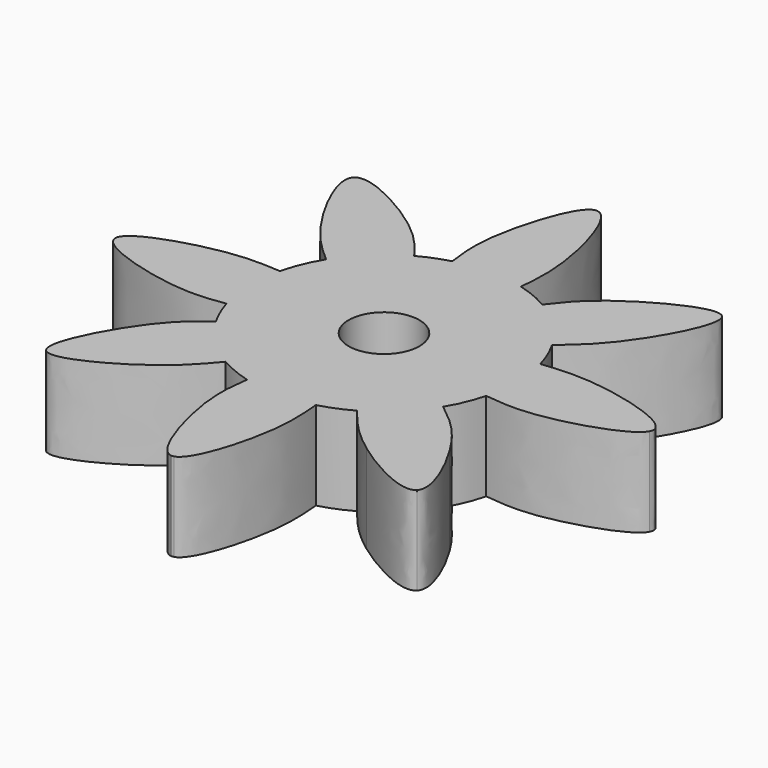
from build123d import *

# Parameters (mm, degrees)
F1_DEPTH = 8
F2_R     = 3.2
F3_DEPTH = 8


with BuildPart() as f1:
    # F0 (on Top) → F1 (new body)
    with BuildSketch(Plane.XY):
        with BuildLine():
            ThreePointArc((11.624215505, -2.9795324957), (11.905683224, -1.5015681703), (12, 0))
            ThreePointArc((12, 0), (11.8901027427, 1.6203261298), (11.5624238722, 3.2109740268))
            ThreePointArc((11.5624238722, 3.2109740268), (11.0655860548, 4.6424998939), (10.3923048454, 6))
            ThreePointArc((10.3923048454, 6), (8.4852813742, 8.4852813742), (6, 10.3923048454))
            ThreePointArc((6, 10.3923048454), (4.5922011884, 11.0865543901), (3.1058285412, 11.5911099155))
            ThreePointArc((3.1058285412, 11.5911099155), (0, 12), (-3.1058285412, 11.5911099155))
            ThreePointArc((-3.1058285412, 11.5911099155), (-4.4398668676, 11.1484340693), (-5.7129920656, 10.5528063404))
            ThreePointArc((-5.7129920656, 10.5528063404), (-8.2605500909, 8.7042123248), (-10.2397735662, 6.25675933))
            ThreePointArc((-10.2397735662, 6.25675933), (-11.0868366823, 4.5915196156), (-11.6651564764, 2.8149821281))
            ThreePointArc((-11.6651564764, 2.8149821281), (-11.9958792367, -0.3144540322), (-11.5016563593, -3.4222654765))
            ThreePointArc((-11.5016563593, -3.4222654765), (-11.0225933032, -4.7436733522), (-10.3923048454, -6))
            ThreePointArc((-10.3923048454, -6), (-8.4852813742, -8.4852813742), (-6, -10.3923048454))
            ThreePointArc((-6, -10.3923048454), (-4.5922011884, -11.0865543901), (-3.1058285412, -11.5911099155))
            ThreePointArc((-3.1058285412, -11.5911099155), (0, -12), (3.1058285412, -11.5911099155))
            ThreePointArc((3.1058285412, -11.5911099155), (4.5432719603, -11.1066952733), (5.908120799, -10.4448125222))
            ThreePointArc((5.908120799, -10.4448125222), (8.3736459378, -8.5954670442), (10.2868074238, -6.1791255875))
            ThreePointArc((10.2868074238, -6.1791255875), (11.0717017858, -4.6278958032), (11.624215505, -2.9795324957))
        make_face()
        with BuildLine():
            ThreePointArc((11.5624238722, 3.2109740268), (11.8901027427, 1.6203261298), (12, 0))
            ThreePointArc((12, 0), (11.905683224, -1.5015681703), (11.624215505, -2.9795324957))
            add(Edge.make_bspline(
                [(11.624215505, -2.9795324957), (13.0711119373, -3.1474625085), (16.2215938385, -3.5354098028), (23.3430398074, -1.2147893088), (23.9974502807, -0.0193380728)],
                knots=[0, 0, 0, 0, 0.2260964002, 0.4754769354, 0.4754769354, 0.4754769354, 0.4754769354], degree=3))
            add(Edge.make_bspline(
                [(23.9974502807, -0.0193380728), (24.0614185813, 0.0975166951), (24.4699625306, 1.4775409149), (16.7275018212, 3.7524414462), (13.1935231835, 3.38198653), (11.5624238722, 3.2109740268)],
                knots=[0.4754769354, 0.4754769354, 0.4754769354, 0.4754769354, 0.4998537595, 0.763872081, 1, 1, 1, 1], degree=3))
        make_face()
        with BuildLine():
            ThreePointArc((6, 10.3923048454), (8.4852813742, 8.4852813742), (10.3923048454, 6))
            add(Edge.make_bspline(
                [(17.0919170156, 16.8124119108), (17.6837825023, 15.7350104435), (14.233378626, 9.2275146766), (11.6451903674, 7.0527541624), (10.3923048454, 6)],
                knots=[0.5132748066, 0.5132748066, 0.5132748066, 0.5132748066, 0.7643869429, 1, 1, 1, 1], degree=3))
            Line((17.0919170156, 16.8124119108), (16.9705629685, 16.9705635618))
            Line((16.9705629685, 16.9705635618), (16.8722269652, 17.046019431))
            add(Edge.make_bspline(
                [(6, 10.3923048454), (6.8772705646, 11.5415832454), (8.7951195762, 14.0540834163), (15.7764959515, 17.7301129885), (16.8722269652, 17.046019431)],
                knots=[0, 0, 0, 0, 0.2244243513, 0.4906263104, 0.4906263104, 0.4906263104, 0.4906263104], degree=3))
        make_face()
        with BuildLine():
            add(Edge.make_bspline(
                [(10.2868074238, -6.1791255875), (11.4270677634, -7.0822286351), (12.865925877, -8.1262783159), (14.5581234006, -10.6857585266), (14.8109868504, -11.0946847194)],
                knots=[0, 0, 0, 0, 0.2257806982, 0.2662434003, 0.2662434003, 0.2662434003, 0.2662434003], degree=3))
            ThreePointArc((10.2868074238, -6.1791255875), (8.3736459378, -8.5954670442), (5.908120799, -10.4448125222))
            add(Edge.make_bspline(
                [(7.0890186874, -11.8532565288), (6.6610674582, -11.3742973278), (6.2831423621, -10.9076828022), (5.908120799, -10.4448125222)],
                knots=[0.9142291133, 0.9142291133, 0.9142291133, 0.9142291133, 1, 1, 1, 1], degree=3))
            add(Edge.make_bspline(
                [(10.0568733092, -14.5338657298), (8.7441655127, -13.5714120718), (7.8396400458, -12.6933452624), (7.0890186874, -11.8532565288)],
                knots=[0.7637879996, 0.7637879996, 0.7637879996, 0.7637879996, 0.9142291133, 0.9142291133, 0.9142291133, 0.9142291133], degree=3))
            add(Edge.make_bspline(
                [(16.8059917931, -17.2725248103), (15.9222786098, -18.1709296498), (12.3524907209, -16.2134042482), (10.0568733491, -14.5338657589)],
                knots=[0.50038259, 0.50038259, 0.50038259, 0.50038259, 0.7648987347, 0.7648987347, 0.7648987347, 0.7648987347], degree=3))
            add(Edge.make_bspline(
                [(14.8109868504, -11.0946847194), (16.2696513341, -13.4536105124), (17.584874947, -16.4762614942), (16.8059918085, -17.2725247947)],
                knots=[0.2662434003, 0.2662434003, 0.2662434003, 0.2662434003, 0.4996559651, 0.4996559651, 0.4996559651, 0.4996559651], degree=3))
        make_face()
        with BuildLine():
            ThreePointArc((-3.1058285412, 11.5911099155), (0, 12), (3.1058285412, 11.5911099155))
            add(Edge.make_bspline(
                [(0.1976441975, 23.9739796614), (1.3779926102, 23.6306464061), (3.5396801636, 16.5893546652), (3.2473427828, 13.2214433713), (3.1058285412, 11.5911099155)],
                knots=[0.5132751075, 0.5132751075, 0.5132751075, 0.5132751075, 0.7643869429, 1, 1, 1, 1], degree=3))
            Line((0.1976441975, 23.9739796614), (0, 24))
            Line((0, 24), (-0.1228977193, 23.9838202083))
            add(Edge.make_bspline(
                [(-3.1058285412, 11.5911099155), (-3.2981671262, 13.0240964307), (-3.7186485167, 16.1568228295), (-1.3814211537, 23.6927333107), (-0.1228977193, 23.9838202083)],
                knots=[0, 0, 0, 0, 0.2244243513, 0.4906257542, 0.4906257542, 0.4906257542, 0.4906257542], degree=3))
        make_face()
        with BuildLine():
            add(Edge.make_bspline(
                [(0.1976441576, -23.973979673), (1.377992585, -23.6306464881), (3.5396801653, -16.5893546847), (3.2473427828, -13.2214433713), (3.1058285412, -11.5911099155)],
                knots=[0.5132751047, 0.5132751047, 0.5132751047, 0.5132751047, 0.7643869429, 1, 1, 1, 1], degree=3))
            ThreePointArc((3.1058285412, -11.5911099155), (0, -12), (-3.1058285412, -11.5911099155))
            add(Edge.make_bspline(
                [(-3.1058285412, -11.5911099155), (-3.2981671262, -13.0240964307), (-3.7186490047, -16.1568264655), (-1.3814157282, -23.6927508039), (-0.1228896428, -23.9838220763)],
                knots=[0, 0, 0, 0, 0.2244243513, 0.4906263236, 0.4906263236, 0.4906263236, 0.4906263236], degree=3))
            Line((-0.1228896428, -23.9838220763), (-4.148e-07, -24.0000007501))
            Line((-4.148e-07, -24.0000007501), (0.1976441576, -23.973979673))
        make_face()
        with BuildLine():
            ThreePointArc((-10.2397735662, 6.25675933), (-8.2605500909, 8.7042123248), (-5.7129920656, 10.5528063404))
            add(Edge.make_bspline(
                [(-5.7129920656, 10.5528063404), (-6.5580524828, 11.7016423726), (-8.4819019469, 14.2776873778), (-19.355634282, 20.2151241331), (-13.9818005189, 9.5546934951), (-11.4637192896, 7.323104241), (-10.2397735662, 6.25675933)],
                knots=[0.0036068796, 0.0036068796, 0.0036068796, 0.0036068796, 0.2249803905, 0.5005320337, 0.7662808066, 1, 1, 1, 1], degree=3))
        make_face()
        with BuildLine():
            add(Edge.make_bspline(
                [(-16.8124081104, -17.0919191033), (-15.7350025484, -17.6837783162), (-9.2275133574, -14.233377056), (-7.0527541624, -11.6451903674), (-6, -10.3923048454)],
                knots=[0.5132751019, 0.5132751019, 0.5132751019, 0.5132751019, 0.7643869429, 1, 1, 1, 1], degree=3))
            ThreePointArc((-6, -10.3923048454), (-8.4852813742, -8.4852813742), (-10.3923048454, -6))
            add(Edge.make_bspline(
                [(-10.3923048454, -6), (-11.5415832454, -6.8772705646), (-14.0540805975, -8.7951174246), (-17.7301047401, -15.7764802864), (-17.0460236746, -16.8722201681)],
                knots=[0, 0, 0, 0, 0.2244243513, 0.4906257599, 0.4906257599, 0.4906257599, 0.4906257599], degree=3))
            Line((-17.0460236746, -16.8722201681), (-16.9705627437, -16.9705627678))
            Line((-16.9705627437, -16.9705627678), (-16.8124081104, -17.0919191033))
        make_face()
        with BuildLine():
            ThreePointArc((-11.5016563593, -3.4222654765), (-11.9958792367, -0.3144540322), (-11.6651564764, 2.8149821281))
            add(Edge.make_bspline(
                [(-11.5016563593, -3.4222654765), (-12.9115656206, -3.6370683177), (-16.0934458137, -4.0981863914), (-27.9807827448, -0.6079790505), (-16.6428417959, 3.1311619375), (-13.2845908531, 2.9264195891), (-11.6651564764, 2.8149821281)],
                knots=[0.0036068808, 0.0036068808, 0.0036068808, 0.0036068808, 0.2249823253, 0.5005363381, 0.7662873964, 1, 1, 1, 1], degree=3))
        make_face()
    extrude(amount=F1_DEPTH)

    # F2 (on Top) → F3 (cut)
    with BuildSketch(Plane.XY):
        Circle(F2_R)
    extrude(amount=F3_DEPTH, mode=Mode.SUBTRACT)


solid = f1.part
